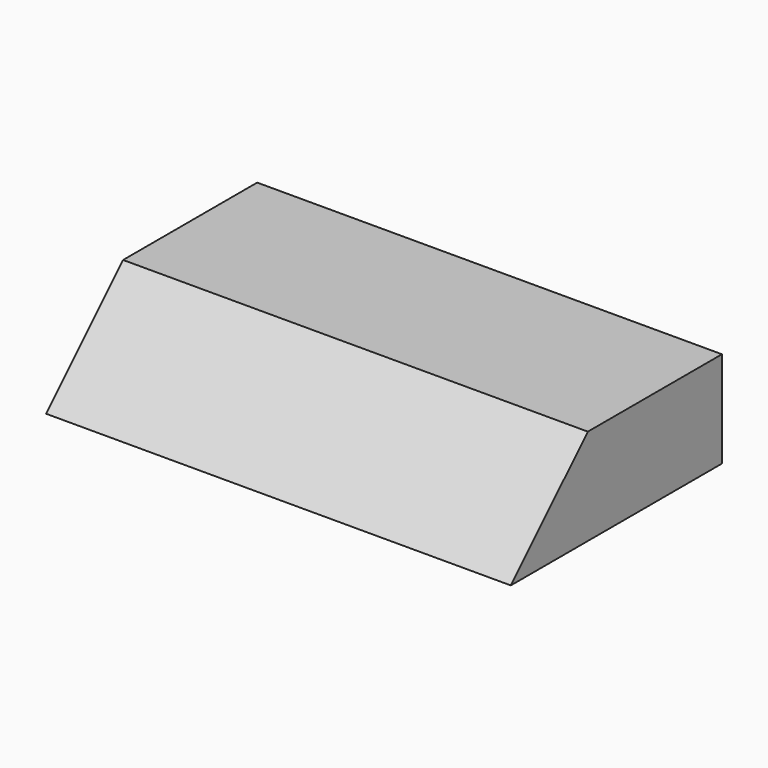
from build123d import *

# Parameters (mm, degrees)
F0_W        = 68.6730742455
F0_H        = 40.0050021708
F1_DEPTH    = 14.224
F2_T1_DEPTH = 147.0579717187


# Not quite as in the source:
# - a fillet or chamfer that OpenCascade refuses, or shapes differently, is made with other operations: its cross-section is extruded or revolved along the edge and cut away or added


with BuildPart() as f1:
    # F0 (on Top) → F1 (new body)
    with BuildSketch(Plane.XY):
        Rectangle(F0_W, F0_H)
    extrude(amount=F1_DEPTH)

    # F2: chamfer of 15.24 on 1 edges, made by hand

    # F2_s2 → F2_t1 (cut)
    with BuildSketch(Plane.YZ.offset(-73.5289858593)):
        Polygon((-20.0025010854, -1.016), (-4.7625010854, 14.224), (-20.0025010854, 14.224), align=None)
    extrude(amount=F2_T1_DEPTH, mode=Mode.SUBTRACT)


solid = f1.part
